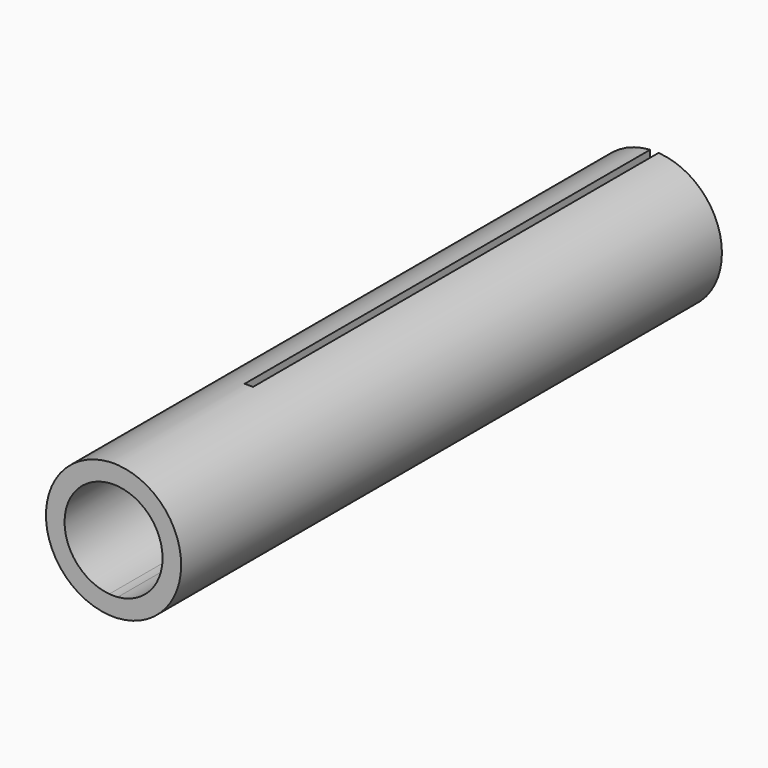
from build123d import *

# Parameters (mm, degrees)
F1_DEPTH = 30
F2_DEPTH = 10
F3_SIZE  = 0.5


with BuildPart() as f1:
    # F0 (on Front) → F1 (new body)
    with BuildSketch(Plane.XZ):
        with BuildLine():
            Line((-0.25, 2.8892040426), (-0.25, 3.9921798557))
            ThreePointArc((-0.25, 3.9921798557), (-4, 0), (-0.25, -3.9921798557))
            Line((-0.25, -3.9921798557), (-0.25, -2.8892040426))
            ThreePointArc((-0.25, -2.8892040426), (-2.9, 0), (-0.25, 2.8892040426))
        make_face()
    extrude(amount=-F1_DEPTH)



with BuildPart() as f1b:
    # F0 (on Front) → F1, piece 2 (new body)
    with BuildSketch(Plane.XZ):
        with BuildLine():
            ThreePointArc((0.25, -3.9921798557), (2.9154759474, -2.7386127875), (4, 0))
            ThreePointArc((4, 0), (2.9154759474, 2.7386127875), (0.25, 3.9921798557))
            Line((0.25, 3.9921798557), (0.25, 2.8892040426))
            ThreePointArc((0.25, 2.8892040426), (2.1371710273, 1.9602295784), (2.9, 0))
            ThreePointArc((2.9, 0), (2.1371710273, -1.9602295784), (0.25, -2.8892040426))
            Line((0.25, -2.8892040426), (0.25, -3.9921798557))
        make_face()
    extrude(amount=-F1_DEPTH)


with BuildPart() as f1_1:
    add(f1.part)

    add(f1b.part)  # F2 merges F1b
    # F0 (on Front) → F2 (join)
    with BuildSketch(Plane.XZ):
        with BuildLine():
            ThreePointArc((0.25, -3.9921798557), (2.9154759474, -2.7386127875), (4, 0))
            ThreePointArc((4, 0), (2.9154759474, 2.7386127875), (0.25, 3.9921798557))
            Line((0.25, 3.9921798557), (0.25, 2.8892040426))
            ThreePointArc((0.25, 2.8892040426), (2.1371710273, 1.9602295784), (2.9, 0))
            ThreePointArc((2.9, 0), (2.1371710273, -1.9602295784), (0.25, -2.8892040426))
            Line((0.25, -2.8892040426), (0.25, -3.9921798557))
        make_face()
        with BuildLine():
            Line((0.25, 2.8892040426), (0.25, 3.9921798557))
            ThreePointArc((0.25, 3.9921798557), (0, 4), (-0.25, 3.9921798557))
            Line((-0.25, 3.9921798557), (-0.25, 2.8892040426))
            ThreePointArc((-0.25, 2.8892040426), (0, 2.9), (0.25, 2.8892040426))
        make_face()
        with BuildLine():
            ThreePointArc((-0.25, -3.9921798557), (0, -4), (0.25, -3.9921798557))
            Line((0.25, -3.9921798557), (0.25, -2.8892040426))
            ThreePointArc((0.25, -2.8892040426), (0, -2.9), (-0.25, -2.8892040426))
            Line((-0.25, -2.8892040426), (-0.25, -3.9921798557))
        make_face()
        with BuildLine():
            Line((-0.25, 2.8892040426), (-0.25, 3.9921798557))
            ThreePointArc((-0.25, 3.9921798557), (-4, 0), (-0.25, -3.9921798557))
            Line((-0.25, -3.9921798557), (-0.25, -2.8892040426))
            ThreePointArc((-0.25, -2.8892040426), (-2.9, 0), (-0.25, 2.8892040426))
        make_face()
    extrude(amount=F2_DEPTH)

    # F3
    f3_edges = [f1_1.edges().sort_by_distance(p)[0] for p in [
        (-2.9, 30, 0),
        (2.9, 30, 0),
    ]]
    chamfer(f3_edges, length=F3_SIZE)


solid = f1_1.part
